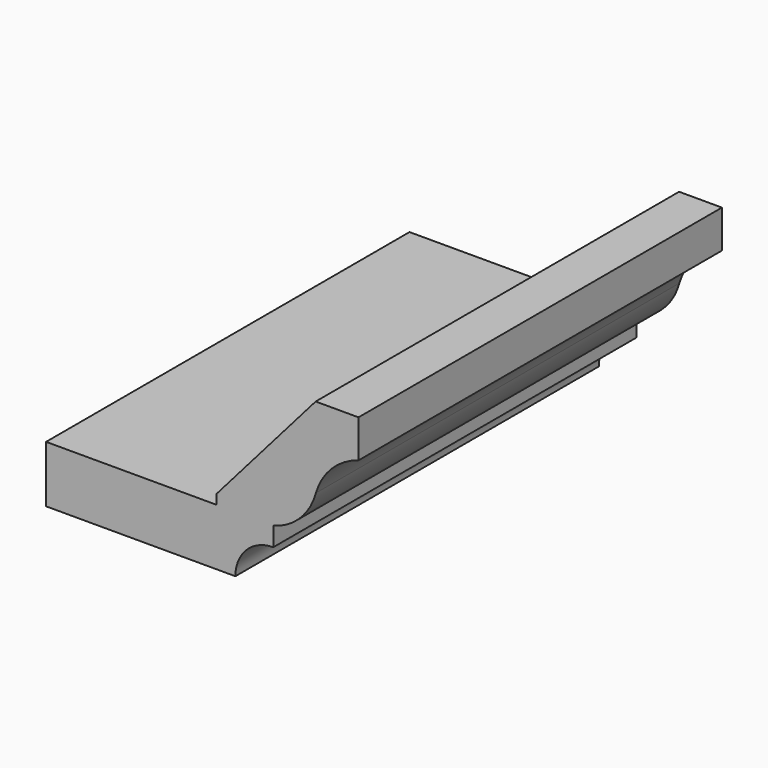
from build123d import *

# Parameters (mm, degrees)
F0_W     = 57.15
F0_H     = 19.05
F1_DEPTH = 152.4


# Not quite as in the source:
# - ends of sketch curves that miss each other by under 0.0002 mm in the source are joined


with BuildPart() as f1:
    # F0 (on Front) → F1 (new body)
    with BuildSketch(Plane.XZ):
        with BuildLine():
            Line((4.745863, -11.1335566), (4.745863, -30.1835566))
            Line((4.745863, -30.1835566), (11.100308, -30.1835566))
            ThreePointArc((11.100308, -30.1835566), (14.8226482602, -21.1970322602), (23.8091726, -17.474692))
            Line((23.8091726, -17.474692), (23.8091726, -11.120247))
            ThreePointArc((23.8091726, -11.120247), (32.8666183043, -5.8802359043), (38.1066276666, 3.1772102678))
            ThreePointArc((38.1066276666, 3.1772102678), (43.4430736289, 12.1382508388), (52.4041076698, 17.4747052267))
            Line((52.4041076698, 17.4747052267), (52.4041116, 30.1835566))
            Line((52.4041116, 30.1835566), (38.0344934, 30.1835566))
            Line((38.0344934, 30.1835566), (4.745863, -7.9430372))
            Line((4.745863, -7.9430372), (4.745863, -11.1335566))
        make_face()
        with Locations((-23.829137, -20.6585566)):
            Rectangle(F0_W, F0_H)
    extrude(amount=F1_DEPTH)


solid = f1.part
